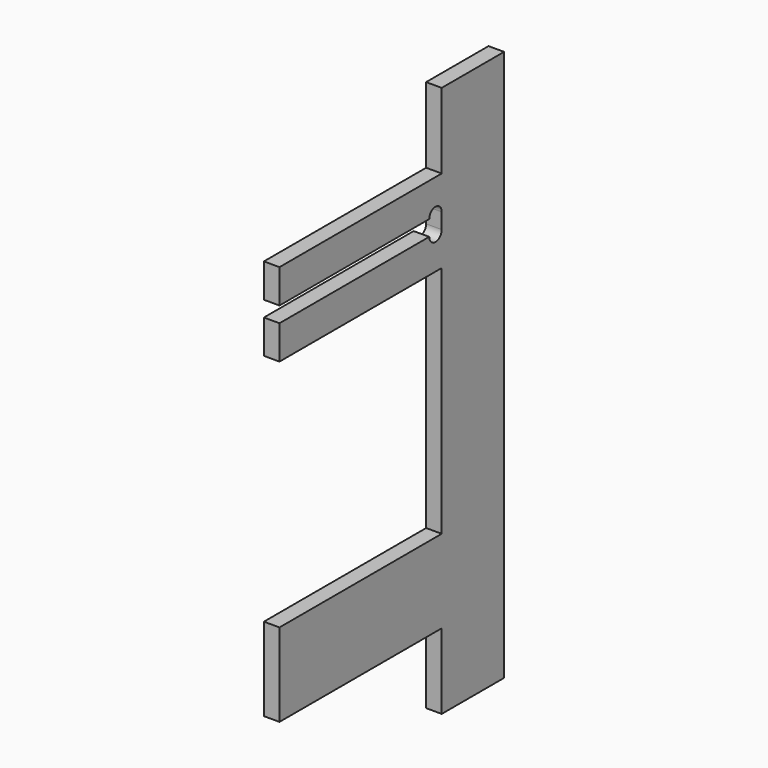
from build123d import *

# Parameters (mm, degrees)
F2_DEPTH = 19.05
F3_W     = 247.65
F3_H     = 19.05
F4_DEPTH = 25.4
F6_DEPTH = 25.4


# Not quite as in the source:
# - a variable given as a bare number and used for a length is read in inches; the dataset says mm whatever the document's units were


with BuildPart() as f2:
    # F1 (on Right) → F2 (new body)
    with BuildSketch(Plane.YZ):
        Polygon((-47.625, 142.875), (-47.625, 0), (-47.625, -142.875), (-295.275, -142.875), (-295.275, -244.475), (-47.625, -244.475), (-47.625, -336.55), (47.625, -336.55), (47.625, 0), (47.625, 336.55), (-47.625, 336.55), (-47.625, 244.475), (-295.275, 244.475), (-295.275, 142.875), align=None)
    extrude(amount=F2_DEPTH)

    # F3 (on face) → F4 (cut)
    with BuildSketch(Plane.YZ.offset(19.05)):
        with Locations((-171.45, 193.675)):
            Rectangle(F3_W, F3_H)
    extrude(amount=-F4_DEPTH, mode=Mode.SUBTRACT)

    # F5 (on face) → F6 (cut)
    with BuildSketch(Plane.YZ.offset(19.05)):
        with BuildLine():
            Line((-47.625, 184.15), (-47.625, 203.2))
            ThreePointArc((-47.625, 203.2), (-57.15, 212.725), (-66.675, 203.2))
            Line((-66.675, 203.2), (-66.675, 184.15))
            ThreePointArc((-66.675, 184.15), (-57.15, 174.625), (-47.625, 184.15))
        make_face()
    extrude(amount=-F6_DEPTH, mode=Mode.SUBTRACT)


solid = f2.part
